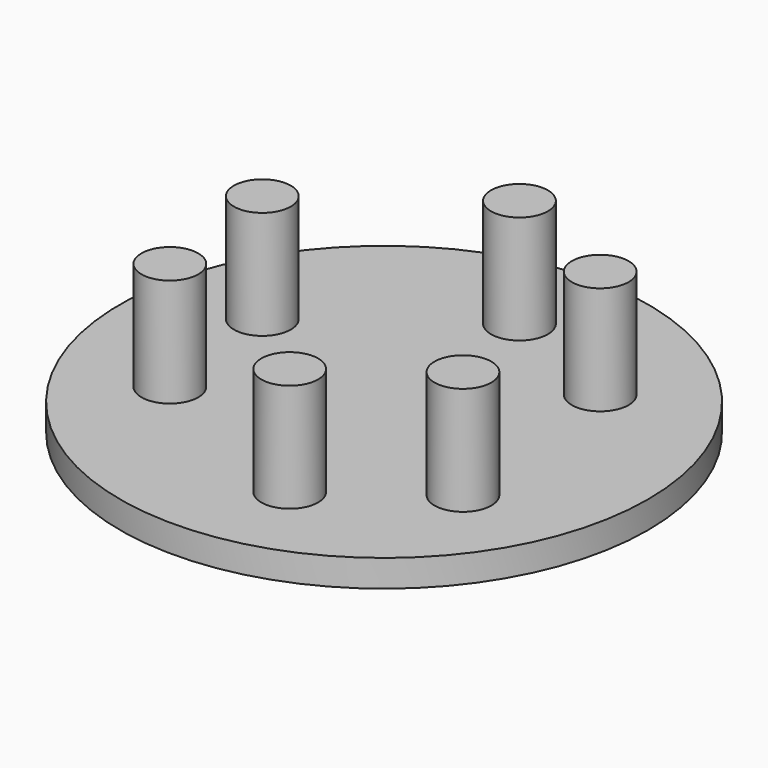
from build123d import *

# Parameters (mm, degrees)
F0_R            = 19.5
F0_R_2          = 2.1
F1_DEPTH        = 2
F2_DEPTH        = 10
F2_COPIES_COUNT = 3


# Not quite as in the source:
# - a pattern or mirror of a feature is missing from the dataset's text; its kind, count and spacing are read off the source's solid


with BuildPart() as f1:
    # F0 (on Top) → F1 (new body)
    with BuildSketch(Plane.XY):
        Circle(F0_R)
        with Locations((9.1651513899, 8.5)):
            Circle(F0_R_2, mode=Mode.SUBTRACT)
        with Locations((0, 12.5)):
            Circle(F0_R_2, mode=Mode.SUBTRACT)
    extrude(amount=F1_DEPTH)

    # F0 (on Top) → F2 (join)
    with BuildSketch(Plane.XY):
        with Locations((0, 12.5)):
            Circle(F0_R_2)
        with Locations((9.1651513899, 8.5)):
            Circle(F0_R_2)
    f2 = extrude(amount=F2_DEPTH)

    # F2_copies: F2 ×3 about axis
    f2_copies_axis = Axis((0, 0, 0), (0, 0, 1))
    for i in range(1, F2_COPIES_COUNT):
        add(f2.rotate(f2_copies_axis, i * 360 / F2_COPIES_COUNT))


solid = f1.part
